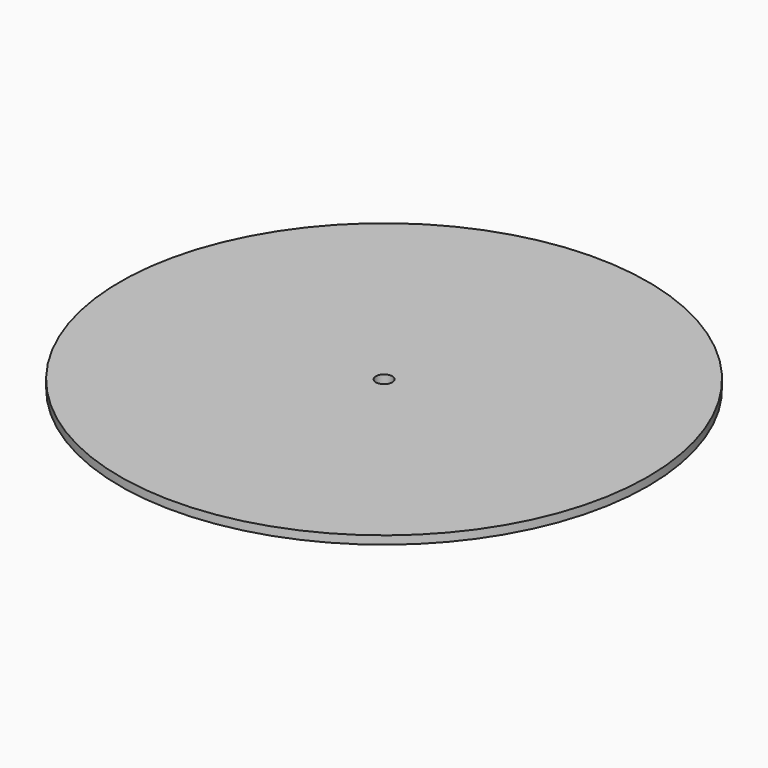
from build123d import *

# Parameters (mm, degrees)
F0_R     = 50.8
F0_R_2   = 6.35
F0_R_3   = 1.5875
F1_DEPTH = 1.5875


# Not quite as in the source:
# - a length typed as a fraction of an inch, garbled in the dataset ("3 / 203.2 mm" for 3/8 in), is restored


with BuildPart() as f1:
    # F0 (on Top) → F1 (new body)
    with BuildSketch(Plane.XY):
        Circle(F0_R)
        Circle(F0_R_2, mode=Mode.SUBTRACT)
        Circle(F0_R_2)
        Circle(F0_R_3, mode=Mode.SUBTRACT)
    extrude(amount=F1_DEPTH)


solid = f1.part
